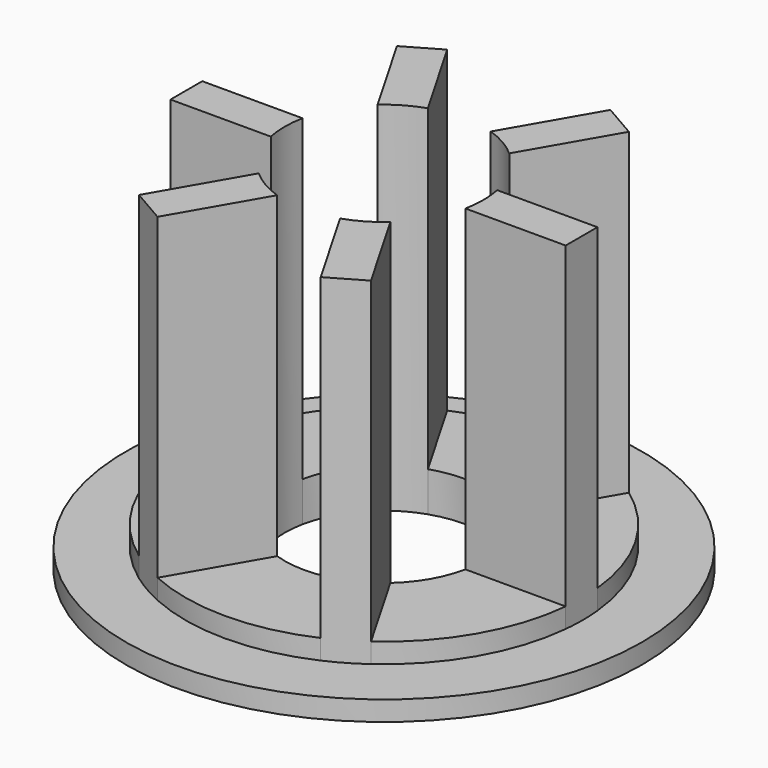
from build123d import *

# Parameters (mm, degrees)
F0_R     = 13
F1_DEPTH = 1
F2_DEPTH = 2
F3_DEPTH = 18


with BuildPart() as f1:
    # F0 (on Top) → F1 (new body)
    with BuildSketch(Plane.XY):
        Circle(F0_R)
        with BuildLine():
            ThreePointArc((9.949874, 1), (9.987461, 0.500628), (10, 0))
            ThreePointArc((10, 0), (9.987461, -0.500628), (9.949874, -1))
            ThreePointArc((9.949874, -1), (8.660254, -5), (5.840963, -8.116844))
            ThreePointArc((5.840963, -8.116844), (5, -8.660254), (4.108912, -9.116844))
            ThreePointArc((4.108912, -9.116844), (0, -10), (-4.108912, -9.116844))
            ThreePointArc((-4.108912, -9.116844), (-5, -8.660254), (-5.840963, -8.116844))
            ThreePointArc((-5.840963, -8.116844), (-8.660254, -5), (-9.949874, -1))
            ThreePointArc((-9.949874, -1), (-10, 0), (-9.949874, 1))
            ThreePointArc((-9.949874, 1), (-8.660254, 5), (-5.840963, 8.116844))
            ThreePointArc((-5.840963, 8.116844), (-5, 8.660254), (-4.108912, 9.116844))
            ThreePointArc((-4.108912, 9.116844), (0, 10), (4.108912, 9.116844))
            ThreePointArc((4.108912, 9.116844), (5, 8.660254), (5.840963, 8.116844))
            ThreePointArc((5.840963, 8.116844), (8.660254, 5), (9.949874, 1))
        make_face(mode=Mode.SUBTRACT)
    extrude(amount=F1_DEPTH)

    # F0 (on Top) → F2 (join)
    with BuildSketch(Plane.XY):
        with BuildLine():
            ThreePointArc((-9.949874, -1), (-8.660254, -5), (-5.840963, -8.116844))
            Line((-5.840963, -8.116844), (-3.315515, -3.742641))
            ThreePointArc((-3.315515, -3.742641), (-4.330127, -2.5), (-4.898979, -1))
            Line((-4.898979, -1), (-9.949874, -1))
        make_face()
        with BuildLine():
            Line((-4.898979, 1), (-9.949874, 1))
            Line((-9.949874, 1), (-9.949874, -1))
            Line((-9.949874, -1), (-4.898979, -1))
            ThreePointArc((-4.898979, -1), (-5, 0), (-4.898979, 1))
        make_face()
        with BuildLine():
            Line((-3.315515, 3.742641), (-5.840963, 8.116844))
            ThreePointArc((-5.840963, 8.116844), (-8.660254, 5), (-9.949874, 1))
            Line((-9.949874, 1), (-4.898979, 1))
            ThreePointArc((-4.898979, 1), (-4.330127, 2.5), (-3.315515, 3.742641))
        make_face()
        with BuildLine():
            Line((-1.583464, 4.742641), (-4.108912, 9.116844))
            Line((-4.108912, 9.116844), (-5.840963, 8.116844))
            Line((-5.840963, 8.116844), (-3.315515, 3.742641))
            ThreePointArc((-3.315515, 3.742641), (-2.5, 4.330127), (-1.583464, 4.742641))
        make_face()
        with BuildLine():
            Line((1.583464, 4.742641), (4.108912, 9.116844))
            ThreePointArc((4.108912, 9.116844), (0, 10), (-4.108912, 9.116844))
            Line((-4.108912, 9.116844), (-1.583464, 4.742641))
            ThreePointArc((-1.583464, 4.742641), (0, 5), (1.583464, 4.742641))
        make_face()
        with BuildLine():
            Line((4.898979, 1), (9.949874, 1))
            ThreePointArc((9.949874, 1), (8.660254, 5), (5.840963, 8.116844))
            Line((5.840963, 8.116844), (3.315515, 3.742641))
            ThreePointArc((3.315515, 3.742641), (4.330127, 2.5), (4.898979, 1))
        make_face()
        with BuildLine():
            Line((9.949874, -1), (9.949874, 1))
            Line((9.949874, 1), (4.898979, 1))
            ThreePointArc((4.898979, 1), (4.974681, 0.502545), (5, 0))
            ThreePointArc((5, 0), (4.974681, -0.502545), (4.898979, -1))
            Line((4.898979, -1), (9.949874, -1))
        make_face()
        with BuildLine():
            Line((3.315515, 3.742641), (5.840963, 8.116844))
            Line((5.840963, 8.116844), (4.108912, 9.116844))
            Line((4.108912, 9.116844), (1.583464, 4.742641))
            ThreePointArc((1.583464, 4.742641), (2.5, 4.330127), (3.315515, 3.742641))
        make_face()
        with BuildLine():
            ThreePointArc((5.840963, -8.116844), (8.660254, -5), (9.949874, -1))
            Line((9.949874, -1), (4.898979, -1))
            ThreePointArc((4.898979, -1), (4.330127, -2.5), (3.315515, -3.742641))
            Line((3.315515, -3.742641), (5.840963, -8.116844))
        make_face()
        with BuildLine():
            Line((4.108912, -9.116844), (5.840963, -8.116844))
            Line((5.840963, -8.116844), (3.315515, -3.742641))
            ThreePointArc((3.315515, -3.742641), (2.5, -4.330127), (1.583464, -4.742641))
            Line((1.583464, -4.742641), (4.108912, -9.116844))
        make_face()
        with BuildLine():
            ThreePointArc((-4.108912, -9.116844), (0, -10), (4.108912, -9.116844))
            Line((4.108912, -9.116844), (1.583464, -4.742641))
            ThreePointArc((1.583464, -4.742641), (0, -5), (-1.583464, -4.742641))
            Line((-1.583464, -4.742641), (-4.108912, -9.116844))
        make_face()
        with BuildLine():
            Line((-5.840963, -8.116844), (-4.108912, -9.116844))
            Line((-4.108912, -9.116844), (-1.583464, -4.742641))
            ThreePointArc((-1.583464, -4.742641), (-2.5, -4.330127), (-3.315515, -3.742641))
            Line((-3.315515, -3.742641), (-5.840963, -8.116844))
        make_face()
    extrude(amount=F2_DEPTH)

    # F0 (on Top) → F3 (join)
    with BuildSketch(Plane.XY):
        with BuildLine():
            Line((3.315515, 3.742641), (5.840963, 8.116844))
            Line((5.840963, 8.116844), (4.108912, 9.116844))
            Line((4.108912, 9.116844), (1.583464, 4.742641))
            ThreePointArc((1.583464, 4.742641), (2.5, 4.330127), (3.315515, 3.742641))
        make_face()
        with BuildLine():
            Line((-1.583464, 4.742641), (-4.108912, 9.116844))
            Line((-4.108912, 9.116844), (-5.840963, 8.116844))
            Line((-5.840963, 8.116844), (-3.315515, 3.742641))
            ThreePointArc((-3.315515, 3.742641), (-2.5, 4.330127), (-1.583464, 4.742641))
        make_face()
        with BuildLine():
            Line((-4.898979, 1), (-9.949874, 1))
            Line((-9.949874, 1), (-9.949874, -1))
            Line((-9.949874, -1), (-4.898979, -1))
            ThreePointArc((-4.898979, -1), (-5, 0), (-4.898979, 1))
        make_face()
        with BuildLine():
            Line((-5.840963, -8.116844), (-4.108912, -9.116844))
            Line((-4.108912, -9.116844), (-1.583464, -4.742641))
            ThreePointArc((-1.583464, -4.742641), (-2.5, -4.330127), (-3.315515, -3.742641))
            Line((-3.315515, -3.742641), (-5.840963, -8.116844))
        make_face()
        with BuildLine():
            Line((4.108912, -9.116844), (5.840963, -8.116844))
            Line((5.840963, -8.116844), (3.315515, -3.742641))
            ThreePointArc((3.315515, -3.742641), (2.5, -4.330127), (1.583464, -4.742641))
            Line((1.583464, -4.742641), (4.108912, -9.116844))
        make_face()
        with BuildLine():
            Line((9.949874, -1), (9.949874, 1))
            Line((9.949874, 1), (4.898979, 1))
            ThreePointArc((4.898979, 1), (4.974681, 0.502545), (5, 0))
            ThreePointArc((5, 0), (4.974681, -0.502545), (4.898979, -1))
            Line((4.898979, -1), (9.949874, -1))
        make_face()
    extrude(amount=F3_DEPTH)


solid = f1.part
